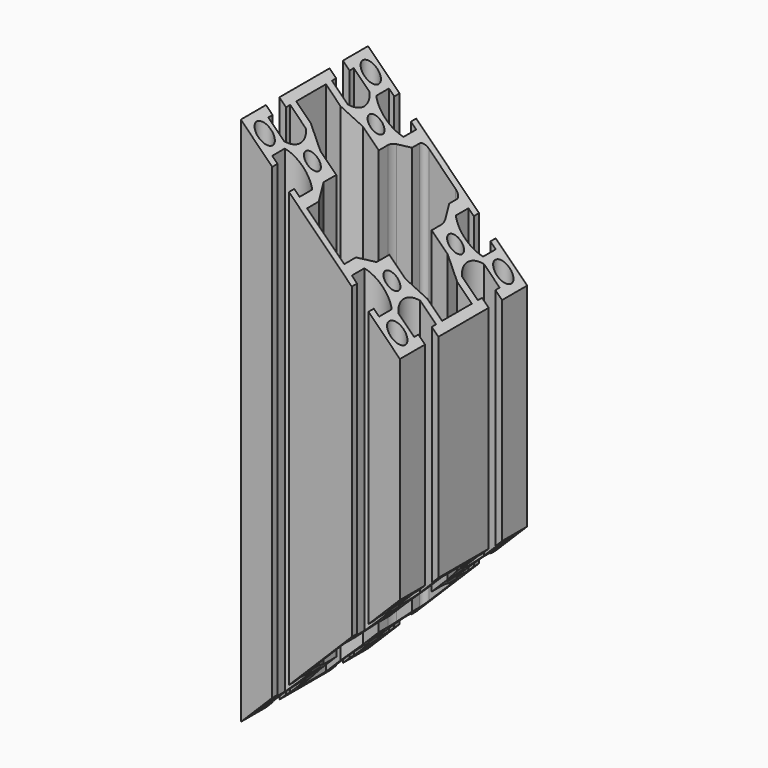
from build123d import *

# Parameters (mm, degrees)
F0_R     = 3
F0_R_2   = 2.5
F1_DEPTH = 200
F2_R     = 2
F3_R     = 7
F5_DEPTH = 60


# Not quite as in the source:
# - a feature names something its author has since deleted; it is built from what else it names


with BuildPart() as f1:
    # F0 (on Top) → F1 (new body)
    with BuildSketch(Plane.XY):
        with BuildLine():
            Line((18.15, -30), (30, -30))
            Line((30, -30), (30, -18.15))
            Line((30, -18.15), (27.5, -18.15))
            Line((27.5, -18.15), (27.5, -20.15))
            Line((27.5, -20.15), (21.5477069044, -20.15))
            ThreePointArc((21.5477069044, -20.15), (19.5, -15), (21.5477069044, -9.85))
            Line((21.5477069044, -9.85), (27.5, -9.85))
            Line((27.5, -9.85), (27.5, -11.85))
            Line((27.5, -11.85), (30, -11.85))
            Line((30, -11.85), (30, 11.85))
            Line((30, 11.85), (27.5, 11.85))
            Line((27.5, 11.85), (27.5, 9.85))
            Line((27.5, 9.85), (21.5477069044, 9.85))
            ThreePointArc((21.5477069044, 9.85), (19.5, 15), (21.5477069044, 20.15))
            Line((21.5477069044, 20.15), (27.5, 20.15))
            Line((27.5, 20.15), (27.5, 18.15))
            Line((27.5, 18.15), (30, 18.15))
            Line((30, 18.15), (30, 30))
            Line((30, 30), (18.15, 30))
            Line((18.15, 30), (18.15, 27.5))
            Line((18.15, 27.5), (20.15, 27.5))
            Line((20.15, 27.5), (20.15, 21.5477069044))
            ThreePointArc((20.15, 21.5477069044), (15, 19.5), (9.85, 21.5477069044))
            Line((9.85, 21.5477069044), (9.85, 27.5))
            Line((9.85, 27.5), (11.85, 27.5))
            Line((11.85, 27.5), (11.85, 30))
            Line((11.85, 30), (-11.85, 30))
            Line((-11.85, 30), (-11.85, 27.5))
            Line((-11.85, 27.5), (-9.85, 27.5))
            Line((-9.85, 27.5), (-9.85, 21.5477069044))
            ThreePointArc((-9.85, 21.5477069044), (-15, 19.5), (-20.15, 21.5477069044))
            Line((-20.15, 21.5477069044), (-20.15, 27.5))
            Line((-20.15, 27.5), (-18.15, 27.5))
            Line((-18.15, 27.5), (-18.15, 30))
            Line((-18.15, 30), (-30, 30))
            Line((-30, 30), (-30, 18.15))
            Line((-30, 18.15), (-27.5, 18.15))
            Line((-27.5, 18.15), (-27.5, 20.15))
            Line((-27.5, 20.15), (-21.5477069044, 20.15))
            ThreePointArc((-21.5477069044, 20.15), (-19.5, 15), (-21.5477069044, 9.85))
            Line((-21.5477069044, 9.85), (-27.5, 9.85))
            Line((-27.5, 9.85), (-27.5, 11.85))
            Line((-27.5, 11.85), (-30, 11.85))
            Line((-30, 11.85), (-30, -11.85))
            Line((-30, -11.85), (-27.5, -11.85))
            Line((-27.5, -11.85), (-27.5, -9.85))
            Line((-27.5, -9.85), (-21.5477069044, -9.85))
            ThreePointArc((-21.5477069044, -9.85), (-19.5, -15), (-21.5477069044, -20.15))
            Line((-21.5477069044, -20.15), (-27.5, -20.15))
            Line((-27.5, -20.15), (-27.5, -18.15))
            Line((-27.5, -18.15), (-30, -18.15))
            Line((-30, -18.15), (-30, -30))
            Line((-30, -30), (-18.15, -30))
            Line((-18.15, -30), (-18.15, -27.5))
            Line((-18.15, -27.5), (-20.15, -27.5))
            Line((-20.15, -27.5), (-20.15, -21.5477069044))
            ThreePointArc((-20.15, -21.5477069044), (-15, -19.5), (-9.85, -21.5477069044))
            Line((-9.85, -21.5477069044), (-9.85, -27.5))
            Line((-9.85, -27.5), (-11.85, -27.5))
            Line((-11.85, -27.5), (-11.85, -30))
            Line((-11.85, -30), (11.85, -30))
            Line((11.85, -30), (11.85, -27.5))
            Line((11.85, -27.5), (9.85, -27.5))
            Line((9.85, -27.5), (9.85, -21.5477069044))
            ThreePointArc((9.85, -21.5477069044), (15, -19.5), (20.15, -21.5477069044))
            Line((20.15, -21.5477069044), (20.15, -27.5))
            Line((20.15, -27.5), (18.15, -27.5))
            Line((18.15, -27.5), (18.15, -30))
        make_face()
        with Locations((-25, -25)):
            Circle(F0_R, mode=Mode.SUBTRACT)
        with Locations((-15, -15)):
            Circle(F0_R_2, mode=Mode.SUBTRACT)
        with Locations((25, -25)):
            Circle(F0_R, mode=Mode.SUBTRACT)
        with Locations((15, -15)):
            Circle(F0_R_2, mode=Mode.SUBTRACT)
        with Locations((-25, 25)):
            Circle(F0_R, mode=Mode.SUBTRACT)
        with Locations((-15, 15)):
            Circle(F0_R_2, mode=Mode.SUBTRACT)
        Polygon((-7, 22), (-7, 27.5), (0, 27.5), (7, 27.5), (7, 22), (10, 16), (10, 10), (16, 10), (22, 7), (27.5, 7), (27.5, 0), (27.5, -7), (22, -7), (16, -10), (10, -10), (10, -16), (7, -22), (7, -27.5), (0, -27.5), (-7, -27.5), (-7, -22), (-10, -16), (-10, -10), (-16, -10), (-22, -7), (-27.5, -7), (-27.5, 0), (-27.5, 7), (-22, 7), (-16, 10), (-10, 10), (-10, 16), align=None, mode=Mode.SUBTRACT)
        with Locations((15, 15)):
            Circle(F0_R_2, mode=Mode.SUBTRACT)
        with Locations((25, 25)):
            Circle(F0_R, mode=Mode.SUBTRACT)
    extrude(amount=F1_DEPTH)

    # F2
    f2_edges = [f1.edges().sort_by_distance(p)[0] for p in [
        (-7, 27.5, 100),
        (7, 27.5, 100),
    ]]
    fillet(f2_edges, radius=F2_R)

    # F3
    f3_edges = [f1.edges().sort_by_distance(p)[0] for p in [
        (-10, 16, 100),
        (10, 16, 100),
    ]]
    fillet(f3_edges, radius=F3_R)

    # F4 (on face) → F5 (cut)
    with BuildSketch(Plane.XZ.offset(30)):
        Polygon((30, 0), (30, 60), (-30, 0), (-18.15, 0), align=None)
        Polygon((30, 140), (30, 200), (-18.15, 200), (-30, 200), align=None)
    extrude(amount=-F5_DEPTH, mode=Mode.SUBTRACT)


solid = f1.part
